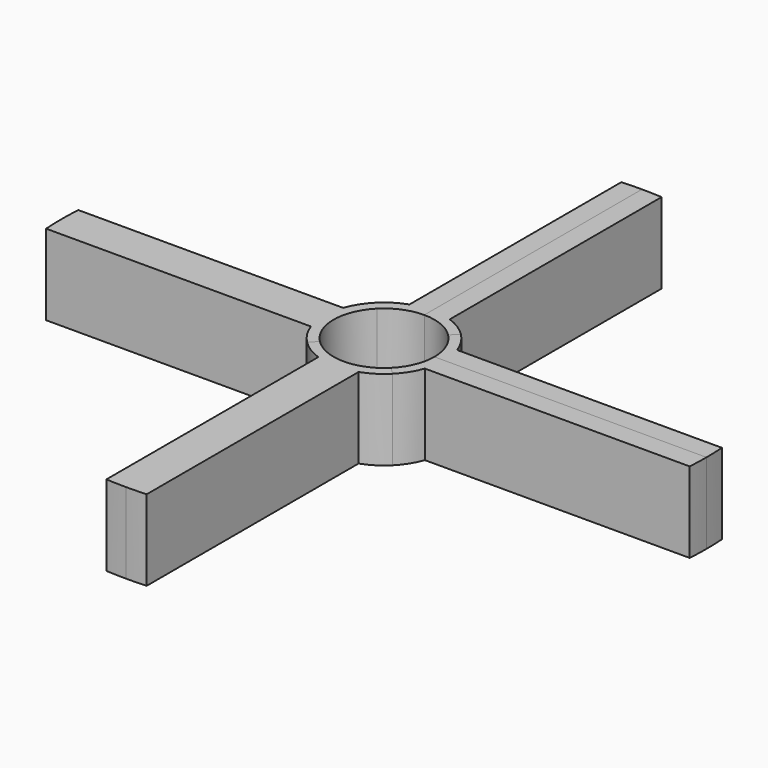
from build123d import *

# Parameters (mm, degrees)
F1_DEPTH        = 25.4
F1_COPIES_COUNT = 4


# Not quite as in the source:
# - a feature of the source that left no trace in its solid (it failed there, or was rolled back) is left out
# - a pattern or mirror of a feature is missing from the dataset's text; its kind, count and spacing are read off the source's solid


with BuildPart() as f1:
    # F0 (on Top) → F1 (new body)
    with BuildSketch(Plane.XY):
        with BuildLine():
            ThreePointArc((-11.2253201513, 11.2253201513), (-6.0750994888, 14.6665875786), (0, 15.875))
            Line((0, 15.875), (0, 101.6))
            ThreePointArc((0, 101.6), (-3.1765529485, 101.5503299422), (-6.35, 101.401368334))
            Line((-6.35, 101.401368334), (-6.35, 17.9605122421))
            ThreePointArc((-6.35, 17.9605122421), (-10.1613099439, 16.1136674976), (-13.4703841816, 13.4703841816))
            Line((-13.4703841816, 13.4703841816), (-11.2253201513, 11.2253201513))
        make_face()
    extrude(amount=F1_DEPTH)


with BuildPart() as f1_copies_1:
    # F1_copies: instance of F1
    add(f1.part.rotate(Axis((0, 0, 0), (0, 0, 1)), 1 * 360 / F1_COPIES_COUNT))


with BuildPart() as f1_copies_2:
    # F1_copies: instance of F1
    add(f1.part.rotate(Axis((0, 0, 0), (0, 0, 1)), 2 * 360 / F1_COPIES_COUNT))


with BuildPart() as f1_copies_3:
    # F1_copies: instance of F1
    add(f1.part.rotate(Axis((0, 0, 0), (0, 0, 1)), 3 * 360 / F1_COPIES_COUNT))


with BuildPart() as f1_1:
    add(f1.part)

    add(f1_copies_1.part)  # F1_copies1 merges F1_copies_1
    # F1_copies1: F1 across plane
    add(f1.part.mirror(Plane(origin=(0, 0, 0), x_dir=(0.7071067812, -0.7071067812, 0), z_dir=(-0.7071067812, -0.7071067812, 0))))



with BuildPart() as f1_2:
    add(f1_1.part)

    add(f1_copies_2.part)  # F4 merges F1_copies_2
    # F4: F1 across plane
    add(f1_1.part.mirror(Plane.XZ))



with BuildPart() as f1_3:
    add(f1_2.part)

    add(f1_copies_3.part)  # F5 merges F1_copies_3
    # F5: F1 across plane
    add(f1_2.part.mirror(Plane.YZ))


solid = f1_3.part
